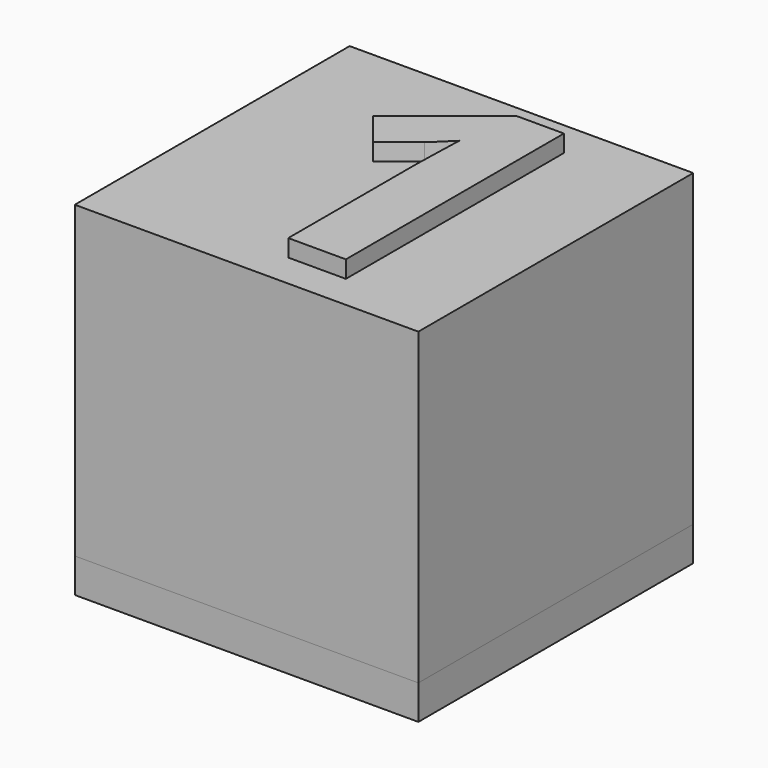
from build123d import *

# Parameters (mm, degrees)
F0_W         = 10
F0_H         = 10
F1_DEPTH     = 10
F2_TEXT_SIZE = 11.1111111111
F3_DEPTH     = 0.5
F4_W         = 5
F4_H         = 1
F5_DEPTH     = 1
F6_W         = 10
F6_H         = 10
F6_W_2       = 5
F6_H_2       = 1
F7_DEPTH     = 1


# Not quite as in the source:
# - Text() gives the source's letters only with a copy of the font that has no kerning and outlines rounded to 1/6400 em; it was checked with that copy


with BuildPart() as f1:
    # F0 (on Top) → F1 (new body)
    with BuildSketch(Plane.XY):
        with Locations((5, 5)):
            Rectangle(F0_W, F0_H)
    extrude(amount=F1_DEPTH)

    # F2 (on face) → F3 (join)
    with BuildSketch(Plane.XY.offset(10)):
        with Locations((2.5, 1)):
            Text('1', F2_TEXT_SIZE, font='Open Sans', font_style=FontStyle.BOLD, text_align=(TextAlign.LEFT, TextAlign.BOTTOM))
    extrude(amount=F3_DEPTH)

    # F4 (on face) → F5 (cut)
    with BuildSketch(Plane(origin=(0, 0, 0), x_dir=(1, 0, 0), z_dir=(0, 0, -1))):
        with Locations((3.9652777778, -5.8888888889)):
            Rectangle(F4_W, F4_H)
    extrude(amount=-F5_DEPTH, mode=Mode.SUBTRACT)


with BuildPart() as f7:
    # F6 (on face) → F7 (new body)
    with BuildSketch(Plane(origin=(0, 0, 0), x_dir=(1, 0, 0), z_dir=(0, 0, -1))):
        with Locations((5, -5)):
            Rectangle(F6_W, F6_H)
        with Locations((3.9652777778, -5.8888888889)):
            Rectangle(F6_W_2, F6_H_2, mode=Mode.SUBTRACT)
    extrude(amount=-F7_DEPTH)


solid = Compound([f1.part, f7.part])
